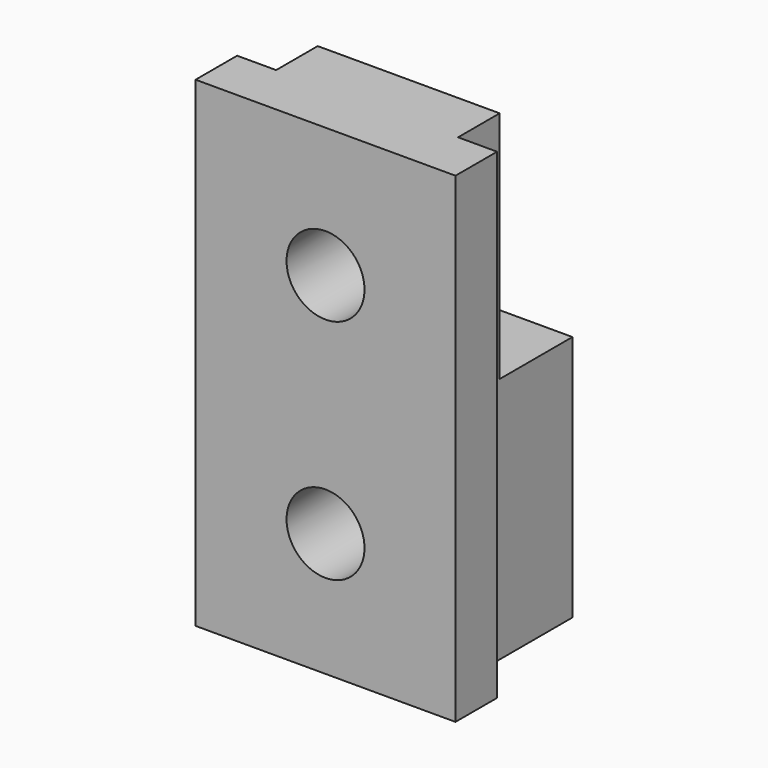
from build123d import *

# Parameters (mm, degrees)
F1_DEPTH = 117.475
F2_W     = 44.45
F2_H     = 60.325
F3_DEPTH = 22.225
F4_R     = 9.525
F5_DEPTH = 25.401
F6_R     = 9.525
F7_DEPTH = 47.626


with BuildPart() as f1:
    # F0 (on Top) → F1 (new body)
    with BuildSketch(Plane.XY):
        Polygon((-41.127444163, -4.0231094092), (-41.127444163, -16.7231094092), (22.372555837, -16.7231094092), (22.372555837, -4.0231094092), (12.847555837, -4.0231094092), (12.847555837, 8.6768905908), (-31.602444163, 8.6768905908), (-31.602444163, -4.0231094092), align=None)
    extrude(amount=F1_DEPTH)

    # F2 (on face) → F3 (join)
    with BuildSketch(Plane(origin=(0, 8.6768905908, 0), x_dir=(-1, 0, 0), z_dir=(0, 1, 0))):
        with Locations((9.377444163, 30.1625)):
            Rectangle(F2_W, F2_H)
    extrude(amount=F3_DEPTH)

    # F4 (on face) → F5 (cut, through all)
    with BuildSketch(Plane(origin=(0, 8.6768905908, 0), x_dir=(-1, 0, 0), z_dir=(0, 1, 0))):
        with Locations((9.377444163, 85.725)):
            Circle(F4_R)
    extrude(amount=-F5_DEPTH, mode=Mode.SUBTRACT)

    # F6 (on face) → F7 (cut, through all)
    with BuildSketch(Plane(origin=(0, 30.9018905908, 0), x_dir=(-1, 0, 0), z_dir=(0, 1, 0))):
        with Locations((9.377444163, 30.1625)):
            Circle(F6_R)
    extrude(amount=-F7_DEPTH, mode=Mode.SUBTRACT)


solid = f1.part
